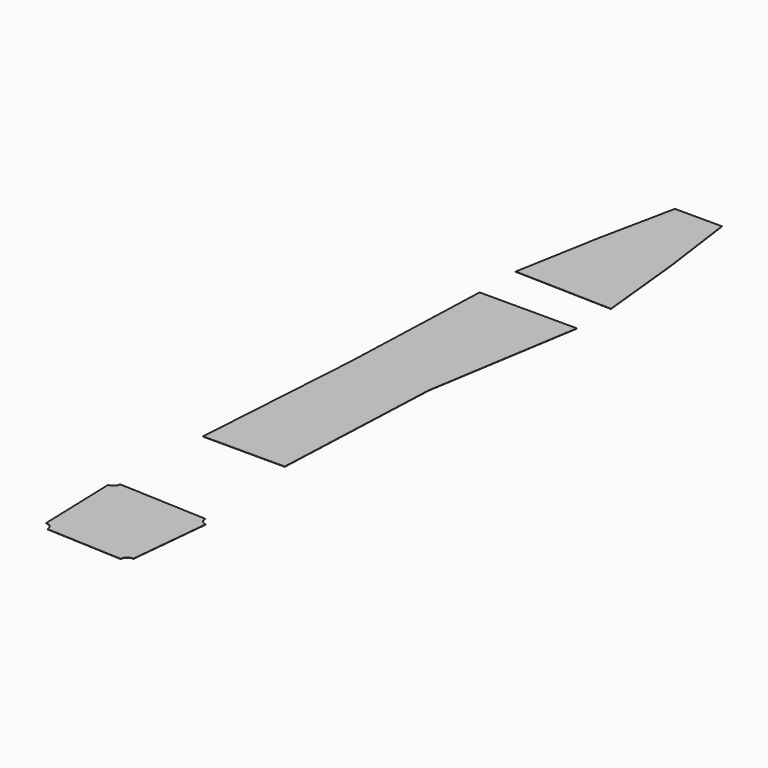
from build123d import *

# Parameters (mm, degrees)
F3_DEPTH = 2
F4_DEPTH = 2
F5_DEPTH = 2


with BuildPart() as f3:
    # F2 (on face) → F3 (new body)
    with BuildSketch(Plane.XY):
        Polygon((-1443.4191744163, 4769.9527426873), (-1783.9887283179, 4769.9527426873), (-1897.4294909214, 4221.6033277621), (-2007.3191407106, 3608.4414445777), (-1302.3924530881, 3588.9879399751), (-1366.9970424155, 4213.0771913099), align=None)
    extrude(amount=F3_DEPTH)


with BuildPart() as f4:
    # F2 (on face) → F4 (new body)
    with BuildSketch(Plane.XY):
        with BuildLine():
            Line((-1482.7704714546, 2165.8153709844), (-1302.6659156704, 3281.5647125244))
            Line((-1302.6659156704, 3281.5647125244), (-2007.3191407106, 3281.5647125244))
            Line((-2007.3191407106, 3281.5647125244), (-2048.7534404071, 2158.4850639998))
            ThreePointArc((-2048.7534404071, 2158.4850639998), (-2048.7850346679, 2157.1314588818), (-2048.8532689015, 2155.7792055394))
            Line((-2048.8532689015, 2155.7792055394), (-2126.8039729209, 938.6436782907))
            ThreePointArc((-2126.8039729209, 938.6436782907), (-2126.7661725299, 937.5217175422), (-2126.753570282, 936.3991909393))
            ThreePointArc((-2126.753570282, 936.3991909393), (-2126.9401190402, 932.0840924022), (-2127.4983732973, 927.8011929161))
            Line((-2127.4983732973, 927.8011929161), (-1535.4920138724, 927.8011929161))
            Line((-1535.4920138724, 927.8011929161), (-1483.2691643821, 2154.1049982133))
            ThreePointArc((-1483.2691643821, 2154.1049982133), (-1483.3641474246, 2159.974848068), (-1482.7704714546, 2165.8153709844))
        make_face()
    extrude(amount=F4_DEPTH)


with BuildPart() as f5:
    # F2 (on face) → F5 (new body)
    with BuildSketch(Plane.XY):
        with BuildLine():
            ThreePointArc((-2126.9499036673, 176.4117163662), (-2141.7820128861, 143.064794042), (-2175.3248371078, 128.6812049348))
            Line((-2175.3248371078, 128.6812049348), (-2156.9079972429, -455.8184208223))
            ThreePointArc((-2156.9079972429, -455.8184208223), (-2120.5391814878, -469.8858711882), (-2105.3333422956, -505.7936192891))
            ThreePointArc((-2105.3333422956, -505.7936192891), (-2105.3473121727, -506.9754790747), (-2105.3892139977, -508.1566784428))
            Line((-2105.3892139977, -508.1566784428), (-1554.1191952458, -534.2394975518))
            ThreePointArc((-1554.1191952458, -534.2394975518), (-1536.8809883486, -498.7829492864), (-1499.3085604422, -486.8399491127))
            Line((-1499.3085604422, -486.8399491127), (-1442.3428307094, 95.664821314))
            ThreePointArc((-1442.3428307094, 95.664821314), (-1475.2571492143, 112.6767149982), (-1487.4259125915, 147.6721159422))
            Line((-1487.4259125915, 147.6721159422), (-2126.9499036673, 176.4117163662))
        make_face()
    extrude(amount=F5_DEPTH)


solid = Compound([f3.part, f4.part, f5.part])
